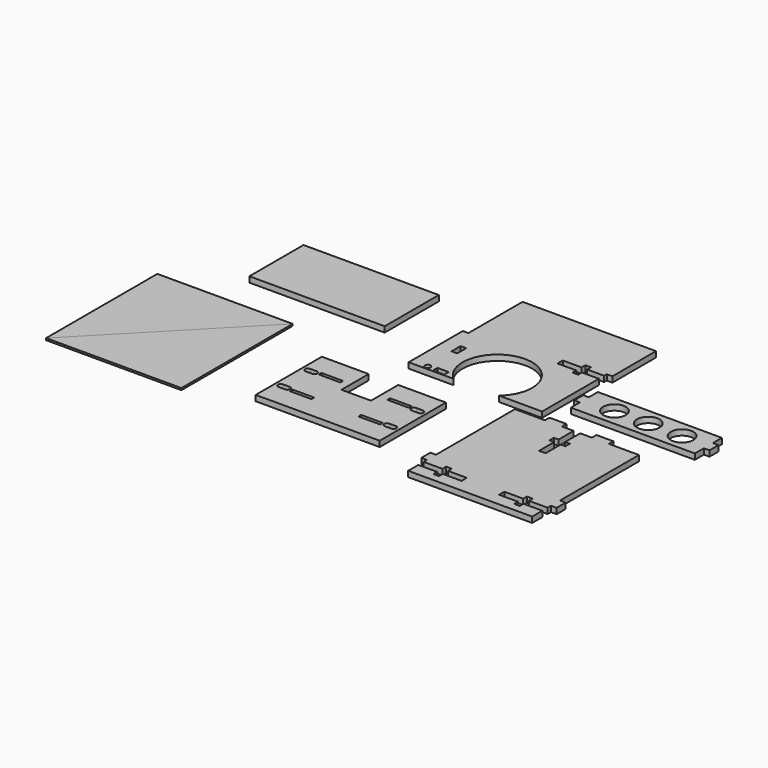
from build123d import *

# Parameters (mm, degrees)
F1_DEPTH  = 3
F2_R      = 18.5
F2_R_2    = 1.5
F2_W      = 6
F2_H      = 3
F2_W_2    = 3
F2_H_2    = 6
F3_DEPTH  = 3
F5_DEPTH  = 3
F6_W      = 11.5
F6_H      = 1.8
F7_DEPTH  = 3
F8_W      = 72
F8_H      = 36
F9_DEPTH  = 3
F11_DEPTH = 3
F13_DEPTH = 1
F14_DEPTH = 1
F15_R     = 6
F16_DEPTH = 3


# Not quite as in the source:
# - a feature names something its author has since deleted; it is built from what else it names


with BuildPart() as f1:
    # F0 (on Top) → F1 (new body)
    with BuildSketch(Plane.XY):
        Polygon((-39.0865747744, 0), (0, 0), (31.9134252256, 0), (31.9134252256, 36), (34.9134252256, 36), (34.9134252256, 72), (-36.0865747744, 72), (-36.0865747744, 36), (-39.0865747744, 36), align=None)
    extrude(amount=F1_DEPTH)

    # F2 (on face) → F3 (cut, through all)
    with BuildSketch(Plane.XY):
        with Locations((-3.0865747744, 14)):
            Circle(F2_R)
        with Locations((-30.5865747744, 2)):
            Circle(F2_R_2)
        with Locations((-23.5865747744, 2)):
            Rectangle(F2_W, F2_H)
        with Locations((-29.8141494989, 21.8136473298)):
            Rectangle(F2_W_2, F2_H_2)
    extrude(amount=F3_DEPTH, mode=Mode.SUBTRACT)

    # F4 (on face) → F5 (cut, through all)
    with BuildSketch(Plane.XY.offset(3)):
        Polygon((31.9134252256, 41.25), (22.9134252256, 41.25), (22.9134252256, 43.75), (19.9134252256, 43.75), (19.9134252256, 41.25), (9.9134252256, 41.25), (9.9134252256, 37.75), (19.9134252256, 37.75), (19.9134252256, 35.25), (22.9134252256, 35.25), (22.9134252256, 37.75), (31.9134252256, 37.75), (31.9134252256, 36), (34.9134252256, 36), (34.9134252256, 43), (31.9134252256, 43), align=None)
    extrude(amount=-F5_DEPTH, mode=Mode.SUBTRACT)


with BuildPart() as f7:
    # F6 (on Top) → F7 (new body)
    with BuildSketch(Plane.XY):
        Polygon((-45.4283840954, -18.6628243396), (-70.3789859414, -18.6628243396), (-70.3789859414, -62.6628243396), (-4.3789859414, -62.6628243396), (-4.3789859414, -18.6628243396), (-29.7082625329, -18.6628243396), (-29.7082625329, -36.7978513241), (-45.4283840954, -36.7978513241), align=None)
        with BuildLine():
            ThreePointArc((-63.8789859414, -48.1628243396), (-62.8183257696, -48.6021641678), (-62.3789859414, -49.6628243396))
            ThreePointArc((-62.3789859414, -49.6628243396), (-62.8183257696, -50.7234845114), (-63.8789859414, -51.1628243396))
            Line((-63.8789859414, -51.1628243396), (-67.3789859414, -51.1628243396))
            ThreePointArc((-67.3789859414, -51.1628243396), (-68.4396461132, -50.7234845114), (-68.8789859414, -49.6628243396))
            ThreePointArc((-68.8789859414, -49.6628243396), (-68.4396461132, -48.6021641678), (-67.3789859414, -48.1628243396))
            Line((-67.3789859414, -48.1628243396), (-63.8789859414, -48.1628243396))
        make_face(mode=Mode.SUBTRACT)
        with Locations((-55.6289859414, -50.2628243396)):
            Rectangle(F6_W, F6_H, mode=Mode.SUBTRACT)
        with Locations((-19.1289859414, -50.2628243396)):
            Rectangle(F6_W, F6_H, mode=Mode.SUBTRACT)
        with BuildLine():
            ThreePointArc((-5.8789859414, -49.6628243396), (-6.3183257696, -50.7234845114), (-7.3789859414, -51.1628243396))
            Line((-7.3789859414, -51.1628243396), (-10.8789859414, -51.1628243396))
            ThreePointArc((-10.8789859414, -51.1628243396), (-11.9396461132, -50.7234845114), (-12.3789859414, -49.6628243396))
            ThreePointArc((-12.3789859414, -49.6628243396), (-11.9396461132, -48.6021641678), (-10.8789859414, -48.1628243396))
            Line((-10.8789859414, -48.1628243396), (-7.3789859414, -48.1628243396))
            ThreePointArc((-7.3789859414, -48.1628243396), (-6.3183257696, -48.6021641678), (-5.8789859414, -49.6628243396))
        make_face(mode=Mode.SUBTRACT)
        with BuildLine():
            ThreePointArc((-68.8789859414, -31.6628243396), (-68.4396461132, -30.6021641678), (-67.3789859414, -30.1628243396))
            Line((-67.3789859414, -30.1628243396), (-63.8789859414, -30.1628243396))
            ThreePointArc((-63.8789859414, -30.1628243396), (-62.8183257696, -30.6021641678), (-62.3789859414, -31.6628243396))
            ThreePointArc((-62.3789859414, -31.6628243396), (-62.8183257696, -32.7234845114), (-63.8789859414, -33.1628243396))
            Line((-63.8789859414, -33.1628243396), (-67.3789859414, -33.1628243396))
            ThreePointArc((-67.3789859414, -33.1628243396), (-68.4396461132, -32.7234845114), (-68.8789859414, -31.6628243396))
        make_face(mode=Mode.SUBTRACT)
        with Locations((-55.6289859414, -31.0628243396)):
            Rectangle(F6_W, F6_H, mode=Mode.SUBTRACT)
        with Locations((-19.1289859414, -31.0628243396)):
            Rectangle(F6_W, F6_H, mode=Mode.SUBTRACT)
        with BuildLine():
            ThreePointArc((-10.8789859414, -33.1628243396), (-11.9396461132, -32.7234845114), (-12.3789859414, -31.6628243396))
            ThreePointArc((-12.3789859414, -31.6628243396), (-11.9396461132, -30.6021641678), (-10.8789859414, -30.1628243396))
            Line((-10.8789859414, -30.1628243396), (-7.3789859414, -30.1628243396))
            ThreePointArc((-7.3789859414, -30.1628243396), (-6.3183257696, -30.6021641678), (-5.8789859414, -31.6628243396))
            ThreePointArc((-5.8789859414, -31.6628243396), (-6.3183257696, -32.7234845114), (-7.3789859414, -33.1628243396))
            Line((-7.3789859414, -33.1628243396), (-10.8789859414, -33.1628243396))
        make_face(mode=Mode.SUBTRACT)
    extrude(amount=F7_DEPTH)


with BuildPart() as f9:
    # F8 (on Top) → F9 (new body)
    with BuildSketch(Plane.XY):
        with Locations((-103.1052859619, 37.0665201917)):
            Rectangle(F8_W, F8_H)
    extrude(amount=F9_DEPTH)


with BuildPart() as f11:
    # F10 (on Top) → F11 (new body)
    with BuildSketch(Plane.XY):
        Polygon((37.7613991201, -5.4026411064), (21.7613991201, -5.4026411064), (21.7613991201, -57.9026411064), (18.7613991201, -57.9026411064), (18.7613991201, -63.9026411064), (21.7613991201, -63.9026411064), (21.7613991201, -66.1526411064), (31.7613991201, -66.1526411064), (31.7613991201, -63.6526411064), (34.7613991201, -63.6526411064), (34.7613991201, -66.1526411064), (44.7613991201, -66.1526411064), (44.7613991201, -69.6526411064), (34.7613991201, -69.6526411064), (34.7613991201, -72.1526411064), (31.7613991201, -72.1526411064), (31.7613991201, -69.6526411064), (21.7613991201, -69.6526411064), (21.7613991201, -76.4026411064), (87.7613991201, -76.4026411064), (87.7613991201, -69.6526411064), (77.7613991201, -69.6526411064), (77.7613991201, -72.1526411064), (74.7613991201, -72.1526411064), (74.7613991201, -69.6526411064), (64.7613991201, -69.6526411064), (64.7613991201, -66.1526411064), (74.7613991201, -66.1526411064), (74.7613991201, -63.6526411064), (77.7613991201, -63.6526411064), (77.7613991201, -66.1526411064), (87.7613991201, -66.1526411064), (87.7613991201, -63.9026411064), (90.7613991201, -63.9026411064), (90.7613991201, -57.9026411064), (87.7613991201, -57.9026411064), (87.7613991201, -5.4026411064), (71.7613991201, -5.4026411064), (71.7613991201, -2.4026411064), (62.7613991201, -2.4026411064), (62.7613991201, -5.4026411064), (56.5113991201, -5.4026411064), (56.5113991201, -15.4026411064), (59.0113991201, -15.4026411064), (59.0113991201, -18.4026411064), (56.5113991201, -18.4026411064), (56.5113991201, -28.4026411064), (53.0113991201, -28.4026411064), (53.0113991201, -18.4026411064), (50.5113991201, -18.4026411064), (50.5113991201, -15.4026411064), (53.0113991201, -15.4026411064), (53.0113991201, -5.4026411064), (46.7613991201, -5.4026411064), (46.7613991201, -2.4026411064), (37.7613991201, -2.4026411064), align=None)
    extrude(amount=F11_DEPTH)


with BuildPart() as f13:
    # F12 (on Top) → F13 (new body)
    with BuildSketch(Plane.XY):
        Polygon((-100.7087475955, -0.1583366255), (-172.7087475955, -0.1583366255), (-172.7087475955, -74.1583366255), align=None)
    extrude(amount=F13_DEPTH)


with BuildPart() as f14:
    # F12 (on Top) → F14 (new body)
    with BuildSketch(Plane.XY):
        Polygon((-100.7087475955, -74.1583366255), (-100.7087475955, -0.1583366255), (-172.7087475955, -74.1583366255), align=None)
    extrude(amount=F14_DEPTH)


with BuildPart() as f16:
    # F15 (on Top) → F16 (new body)
    with BuildSketch(Plane.XY):
        Polygon((36.0482842449, 22.1834971545), (36.0482842449, 16.1834971545), (39.0482842449, 16.1834971545), (39.0482842449, 10.1834971545), (105.0482842449, 10.1834971545), (105.0482842449, 16.1834971545), (108.0482842449, 16.1834971545), (108.0482842449, 22.1834971545), (105.0482842449, 22.1834971545), (105.0482842449, 28.1834971545), (39.0482842449, 28.1834971545), (39.0482842449, 22.1834971545), align=None)
        with Locations((55.0482842449, 19.1834971545)):
            Circle(F15_R, mode=Mode.SUBTRACT)
        with Locations((73.0482842449, 19.1834971545)):
            Circle(F15_R, mode=Mode.SUBTRACT)
        with Locations((91.0482842449, 19.1834971545)):
            Circle(F15_R, mode=Mode.SUBTRACT)
    extrude(amount=F16_DEPTH)


solid = Compound([f1.part, f7.part, f9.part, f11.part, f13.part, f14.part, f16.part])
